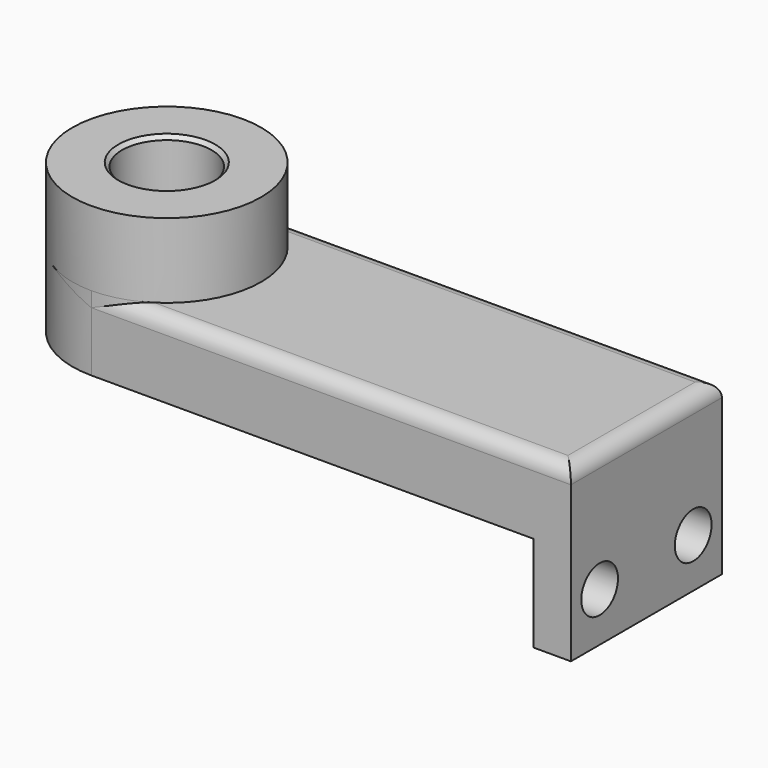
from build123d import *

# Parameters (mm, degrees)
F1_DEPTH     = 25.4
F2_DEPTH     = 50.8
F3_W         = 64.2605721951
F3_H         = 58.0011609286
F3_R         = 7.8158537252
F4_DEPTH     = 12.7
F5_T1_DEPTH  = 89.6605721951
F5_T6_DEPTH  = 197.5881144994
F5_S7_R      = 32.1302860975
F5_T8_DEPTH  = 100
F5_T12_DEPTH = 197.5881144994
F5_S13_R     = 32.1302860975
F5_T14_DEPTH = 100


# Not quite as in the source:
# - a fillet or chamfer that OpenCascade refuses, or shapes differently, is made with other operations: its cross-section is extruded or revolved along the edge and cut away or added


with BuildPart() as f1:
    # F0 (on Top) → F1 (new body)
    with BuildSketch(Plane.XY):
        with BuildLine():
            Line((81.6490572497, -32.1302860975), (81.6490572497, 32.1302860975))
            Line((81.6490572497, 32.1302860975), (-81.6490572497, 32.1302860975))
            ThreePointArc((-81.6490572497, 32.1302860975), (-58.9295140687, 22.719543181), (-49.5187711522, 0))
            ThreePointArc((-49.5187711522, 0), (-58.9295140687, -22.719543181), (-81.6490572497, -32.1302860975))
            Line((-81.6490572497, -32.1302860975), (81.6490572497, -32.1302860975))
        make_face()
        with BuildLine():
            Line((-81.6490572497, 15.24), (-81.6490572497, 32.1302860975))
            ThreePointArc((-81.6490572497, 32.1302860975), (-113.7793433473, 0), (-81.6490572497, -32.1302860975))
            Line((-81.6490572497, -32.1302860975), (-81.6490572497, -15.24))
            ThreePointArc((-81.6490572497, -15.24), (-96.8890572497, 0), (-81.6490572497, 15.24))
        make_face()
        with BuildLine():
            ThreePointArc((-49.5187711522, 0), (-58.9295140687, 22.719543181), (-81.6490572497, 32.1302860975))
            Line((-81.6490572497, 32.1302860975), (-81.6490572497, 15.24))
            ThreePointArc((-81.6490572497, 15.24), (-70.8727499044, 10.7763073453), (-66.4090572497, 0))
            ThreePointArc((-66.4090572497, 0), (-70.8727499044, -10.7763073453), (-81.6490572497, -15.24))
            Line((-81.6490572497, -15.24), (-81.6490572497, -32.1302860975))
            ThreePointArc((-81.6490572497, -32.1302860975), (-58.9295140687, -22.719543181), (-49.5187711522, 0))
        make_face()
    extrude(amount=F1_DEPTH)

    # F0 (on Top) → F2 (join)
    with BuildSketch(Plane.XY):
        with BuildLine():
            Line((-81.6490572497, 15.24), (-81.6490572497, 32.1302860975))
            ThreePointArc((-81.6490572497, 32.1302860975), (-113.7793433473, 0), (-81.6490572497, -32.1302860975))
            Line((-81.6490572497, -32.1302860975), (-81.6490572497, -15.24))
            ThreePointArc((-81.6490572497, -15.24), (-96.8890572497, 0), (-81.6490572497, 15.24))
        make_face()
        with BuildLine():
            ThreePointArc((-49.5187711522, 0), (-58.9295140687, 22.719543181), (-81.6490572497, 32.1302860975))
            Line((-81.6490572497, 32.1302860975), (-81.6490572497, 15.24))
            ThreePointArc((-81.6490572497, 15.24), (-70.8727499044, 10.7763073453), (-66.4090572497, 0))
            ThreePointArc((-66.4090572497, 0), (-70.8727499044, -10.7763073453), (-81.6490572497, -15.24))
            Line((-81.6490572497, -15.24), (-81.6490572497, -32.1302860975))
            ThreePointArc((-81.6490572497, -32.1302860975), (-58.9295140687, -22.719543181), (-49.5187711522, 0))
        make_face()
    extrude(amount=F2_DEPTH)

    # F3 (on face) → F4 (join)
    with BuildSketch(Plane.YZ.offset(81.6490572497)):
        with Locations((0, -3.6005804643)):
            Rectangle(F3_W, F3_H)
        with Locations((-19.9125986546, -15.9243624657)):
            Circle(F3_R, mode=Mode.SUBTRACT)
        with Locations((19.9125986546, -15.9243624657)):
            Circle(F3_R, mode=Mode.SUBTRACT)
    extrude(amount=-F4_DEPTH)

    # F5: fillet of radius 5.08 on 3 edges, made by hand

    # F5_s2 → F5_t1 (cut)
    with BuildSketch(Plane.XZ.offset(-44.8302860975)):
        with BuildLine():
            ThreePointArc((81.6490572497, 20.32), (80.1611596982, 23.9121024484), (76.5690572497, 25.4))
            Line((76.5690572497, 25.4), (81.6490572497, 25.4))
            Line((81.6490572497, 25.4), (81.6490572497, 20.32))
        make_face()
    extrude(amount=F5_T1_DEPTH, mode=Mode.SUBTRACT)


with BuildPart() as f5_tool4:
    # F5_s5 → F5_t6 (new body)
    with BuildSketch(Plane.YZ.offset(94.3490572497)):
        with BuildLine():
            ThreePointArc((-27.0502860975, 25.4), (-30.642388546, 23.9121024484), (-32.1302860975, 20.32))
            Line((-32.1302860975, 20.32), (-32.1302860975, 25.4))
            Line((-32.1302860975, 25.4), (-27.0502860975, 25.4))
        make_face()
    extrude(amount=-F5_T6_DEPTH)

    # F5_s7 → F5_t8 (cut, symmetric)
    with BuildSketch(Plane.XY.offset(22.9)):
        with Locations((-81.6490572497, 0)):
            Circle(F5_S7_R)
    extrude(amount=F5_T8_DEPTH, both=True, mode=Mode.SUBTRACT)


with BuildPart() as f1_1:
    add(f1.part)

    # F5_t3: cut F5_tool4
    add(f5_tool4.part, mode=Mode.SUBTRACT)


with BuildPart() as f5_tool10:
    # F5_s11 → F5_t12 (new body)
    with BuildSketch(Plane.YZ.offset(-103.2390572497)):
        with BuildLine():
            ThreePointArc((32.1302860975, 20.32), (30.642388546, 23.9121024484), (27.0502860975, 25.4))
            Line((27.0502860975, 25.4), (32.1302860975, 25.4))
            Line((32.1302860975, 25.4), (32.1302860975, 20.32))
        make_face()
    extrude(amount=F5_T12_DEPTH)

    # F5_s13 → F5_t14 (cut, symmetric)
    with BuildSketch(Plane.XY.offset(22.9)):
        with Locations((-81.6490572497, 0)):
            Circle(F5_S13_R)
    extrude(amount=F5_T14_DEPTH, both=True, mode=Mode.SUBTRACT)


with BuildPart() as f1_2:
    add(f1_1.part)

    # F5_t9: cut F5_tool10
    add(f5_tool10.part, mode=Mode.SUBTRACT)

    # F6: chamfer of 1.27 on 1 edges, made by hand

    # F6_s1 → F6_t2 (revolve, cut)
    with BuildSketch(Plane.YZ.offset(-81.6490572497)):
        Polygon((15.24, 49.53), (16.51, 50.8), (15.24, 50.8), align=None)
    revolve(axis=Axis((-81.6490572497, 0, 50.8), (0, 0, -1)), mode=Mode.SUBTRACT)


solid = f1_2.part
